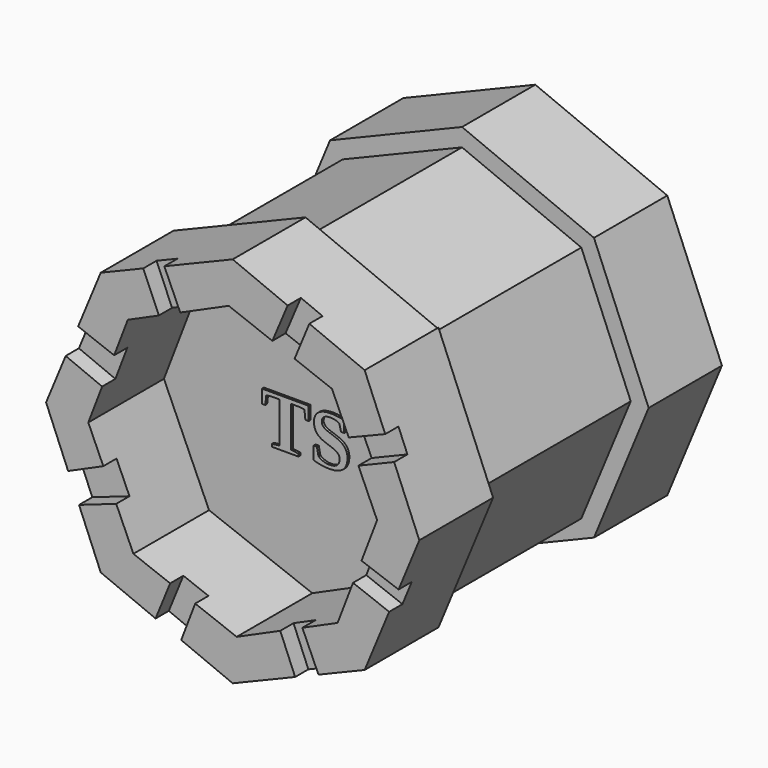
from build123d import *

# Parameters (mm, degrees)
F1_DEPTH      = 20.32
F3_DEPTH      = 5.08
F4_W          = 10.5106048286
F4_H          = 7.6728934978
F5_DEPTH      = 0.889
F6_W          = 7.6728934978
F6_H          = 10.5106048286
F7_DEPTH      = 0.889
F8_W          = 7.6728934978
F8_H          = 10.5106048286
F9_DEPTH      = 0.889
F10_W         = 10.4425107129
F10_H         = 7.6728934978
F11_DEPTH     = 0.889
F12_W         = 10.4425107129
F12_H         = 7.6728934978
F13_DEPTH     = 0.889
F14_W         = 7.6728934978
F14_H         = 10.4425107129
F15_DEPTH     = 0.889
F16_W         = 7.6728934978
F16_H         = 10.4425107129
F17_DEPTH     = 0.889
F18_W         = 10.5106048286
F18_H         = 7.6728934978
F19_DEPTH     = 0.889
F21_DEPTH     = 0.889
F23_DEPTH     = 0.889
F25_DEPTH     = 0.889
F27_DEPTH     = 0.889
F29_DEPTH     = 0.889
F31_DEPTH     = 0.889
F33_DEPTH     = 0.889
F35_DEPTH     = 0.889
F36_TEXT_SIZE = 3.9382759655
F37_DEPTH     = 0.127


# Not quite as in the source:
# - Text() gives the source's letters only with a copy of the font that has no kerning and outlines rounded to 1/6400 em; it was checked with that copy


with BuildPart() as f1:
    # F0 (on Front) → F1 (new body)
    with BuildSketch(Plane.XZ):
        Polygon((7.0888292577, -7.0888292577), (10.0251184776, 0), (7.0888292577, 7.0888292577), (0, 10.0251184776), (-7.0888292577, 7.0888292577), (-10.0251184776, 0), (-7.0888292577, -7.0888292577), (0, -10.0251184776), align=None)
    extrude(amount=F1_DEPTH)

    # F2 (on face) → F3 (cut)
    with BuildSketch(Plane.XZ.offset(20.32)):
        Polygon((7.7576608895, 0.2128587071), (5.3349807858, 5.6360084563), (-0.2128587071, 7.7576608895), (-5.6360084563, 5.3349807858), (-7.7576608895, -0.2128587071), (-5.3349807858, -5.6360084563), (0.2128587071, -7.7576608895), (5.6360084563, -5.3349807858), align=None)
    extrude(amount=-F3_DEPTH, mode=Mode.SUBTRACT)

    # F4 (on face) → F5 (cut)
    with BuildSketch(Plane(origin=(-8.5569738677, 0, 3.5444146289), x_dir=(0, -1, 0), z_dir=(-0.9238795325, 0, 0.3826834324))):
        with Locations((10.176721029, 0)):
            Rectangle(F4_W, F4_H)
    extrude(amount=-F5_DEPTH, mode=Mode.SUBTRACT)

    # F6 (on face) → F7 (cut)
    with BuildSketch(Plane(origin=(-3.5444146289, 0, 8.5569738677), x_dir=(0.9238795325, 0, 0.3826834324), z_dir=(-0.3826834324, 0, 0.9238795325))):
        with Locations((0, -10.176721029)):
            Rectangle(F6_W, F6_H)
    extrude(amount=-F7_DEPTH, mode=Mode.SUBTRACT)

    # F8 (on face) → F9 (cut)
    with BuildSketch(Plane(origin=(3.5444146289, 0, 8.5569738677), x_dir=(0.9238795325, 0, -0.3826834324), z_dir=(0.3826834324, 0, 0.9238795325))):
        with Locations((0, -10.176721029)):
            Rectangle(F8_W, F8_H)
    extrude(amount=-F9_DEPTH, mode=Mode.SUBTRACT)

    # F10 (on face) → F11 (cut)
    with BuildSketch(Plane(origin=(8.5569738677, 0, 3.5444146289), x_dir=(0, 1, 0), z_dir=(0.9238795325, 0, 0.3826834324))):
        with Locations((-10.1426739711, 0)):
            Rectangle(F10_W, F10_H)
    extrude(amount=-F11_DEPTH, mode=Mode.SUBTRACT)

    # F12 (on face) → F13 (cut)
    with BuildSketch(Plane(origin=(8.5569738677, 0, -3.5444146289), x_dir=(0, 1, 0), z_dir=(0.9238795325, 0, -0.3826834324))):
        with Locations((-10.1426739711, 0)):
            Rectangle(F12_W, F12_H)
    extrude(amount=-F13_DEPTH, mode=Mode.SUBTRACT)

    # F14 (on face) → F15 (cut)
    with BuildSketch(Plane(origin=(3.5444146289, 0, -8.5569738677), x_dir=(0.9238795325, 0, 0.3826834324), z_dir=(0.3826834324, 0, -0.9238795325))):
        with Locations((0, 10.1426739711)):
            Rectangle(F14_W, F14_H)
    extrude(amount=-F15_DEPTH, mode=Mode.SUBTRACT)

    # F16 (on face) → F17 (cut)
    with BuildSketch(Plane(origin=(-3.5444146289, 0, -8.5569738677), x_dir=(0.9238795325, 0, -0.3826834324), z_dir=(-0.3826834324, 0, -0.9238795325))):
        with Locations((0, 10.1426739711)):
            Rectangle(F16_W, F16_H)
    extrude(amount=-F17_DEPTH, mode=Mode.SUBTRACT)

    # F18 (on face) → F19 (cut)
    with BuildSketch(Plane(origin=(-8.5569738677, 0, -3.5444146289), x_dir=(0, -1, 0), z_dir=(-0.9238795325, 0, -0.3826834324))):
        with Locations((10.176721029, 0)):
            Rectangle(F18_W, F18_H)
    extrude(amount=-F19_DEPTH, mode=Mode.SUBTRACT)

    # F20 (on face) → F21 (cut)
    with BuildSketch(Plane.XZ.offset(20.32)):
        Polygon((4.1169620036, 8.31981698), (2.951762417, 8.8024584516), (2.1299355635, 6.8617093806), (3.3238668567, 6.40511592), align=None)
    extrude(amount=-F21_DEPTH, mode=Mode.SUBTRACT)

    # F22 (on face) → F23 (cut)
    with BuildSketch(Plane.XZ.offset(20.32)):
        Polygon((8.6745951533, 3.260451726), (8.1924580528, 4.4244336528), (6.2318925298, 3.628278797), (6.7519757635, 2.4640766994), align=None)
    extrude(amount=-F23_DEPTH, mode=Mode.SUBTRACT)

    # F24 (on face) → F25 (cut)
    with BuildSketch(Plane.XZ.offset(20.32)):
        Polygon((8.4053308522, -3.9105132536), (8.9097336882, -2.692777086), (6.9203368696, -1.9766324619), (6.4646005312, -3.168322494), align=None)
    extrude(amount=-F25_DEPTH, mode=Mode.SUBTRACT)

    # F26 (on face) → F27 (cut)
    with BuildSketch(Plane.XZ.offset(20.32)):
        Polygon((-3.6721267161, 8.5040737891), (-4.8033726252, 8.0354963912), (-3.9686209859, 6.0798516887), (-2.8186516312, 6.5935767385), align=None)
    extrude(amount=-F27_DEPTH, mode=Mode.SUBTRACT)

    # F28 (on face) → F29 (cut)
    with BuildSketch(Plane.XZ.offset(20.32)):
        Polygon((-2.0128920811, -6.9064701545), (-3.361127834, -6.390866257), (-4.1440163769, -8.3086106917), (-2.7672070877, -8.878903772), align=None)
    extrude(amount=-F29_DEPTH, mode=Mode.SUBTRACT)

    # F30 (on face) → F31 (cut)
    with BuildSketch(Plane.XZ.offset(20.32)):
        Polygon((3.3533358141, -8.6361213043), (4.484463586, -8.1675928404), (4.6072077905, -8.1167505261), (3.7424096581, -6.1809069256), (2.5559051222, -6.7109533129), align=None)
    extrude(amount=-F31_DEPTH, mode=Mode.SUBTRACT)

    # F32 (on face) → F33 (cut)
    with BuildSketch(Plane.XZ.offset(20.32)):
        Polygon((-7.0148331538, 1.7295372217), (-6.9445106996, 1.9134211051), (-6.3705913131, 3.4141441211), (-8.3045766532, 4.1537554072), (-8.9727886497, 2.5405489427), align=None)
    extrude(amount=-F33_DEPTH, mode=Mode.SUBTRACT)

    # F34 (on face) → F35 (cut)
    with BuildSketch(Plane.XZ.offset(20.32)):
        Polygon((-8.2557426236, -4.2716511837), (-6.2571333464, -3.5717774339), (-6.9518214575, -2.0167237353), (-8.8403147962, -2.8603691165), align=None)
    extrude(amount=-F35_DEPTH, mode=Mode.SUBTRACT)

    # F36 (on face) → F37 (join)
    with BuildSketch(Plane.XZ.offset(15.24)):
        with Locations((-2.4481923326, -1.4573407503)):
            Text('TS', F36_TEXT_SIZE, font='Tinos', font_style=FontStyle.BOLD, text_align=(TextAlign.LEFT, TextAlign.BOTTOM))
    extrude(amount=F37_DEPTH)


solid = f1.part
